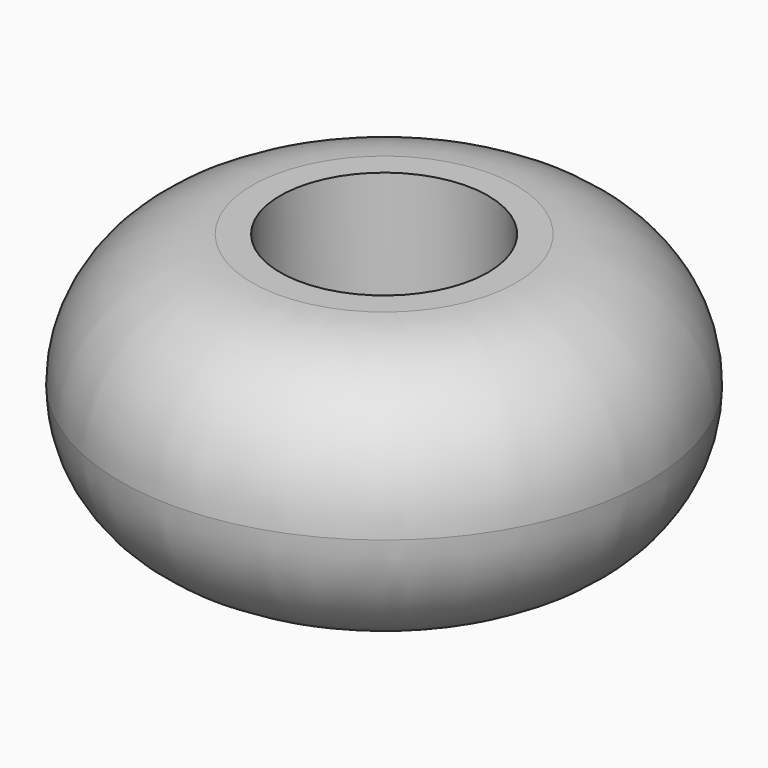
from build123d import *

# Parameters (mm, degrees)
F0_W     = 25.4
F0_H     = 25.4
F2_R     = 12.69999
F3_R     = 10
F4_DEPTH = 20.32
F5_R     = 10


# Not quite as in the source:
# - a fillet or chamfer is up to 0.001 mm smaller than in the source, because OpenCascade refuses the exact size


with BuildPart() as f1:
    # F0 (on Front) → F1 (revolve)
    with BuildSketch(Plane.XZ):
        with Locations((12.7, 12.7)):
            Rectangle(F0_W, F0_H)
    revolve(axis=Axis((0, 0, 17.3243917525), (0, 0, 1)))

    # F2 (radius 12.7 in the source; OpenCascade refuses exactly that, so slightly less here)
    f2_edges = [f1.edges().sort_by_distance(p)[0] for p in [
        (-25.4, 0, 0),
        (-25.4, 0, 25.4),
        (25.4, 0, 12.7),
    ]]
    fillet(f2_edges, radius=F2_R)

    # F3 (on face) → F4 (cut)
    with BuildSketch(Plane.XY.offset(25.4)):
        Circle(F3_R)
    extrude(amount=-F4_DEPTH, mode=Mode.SUBTRACT)

    # F5
    f5_edges = [f1.edges().sort_by_distance(p)[0] for p in [
        (-10, 0, 5.08),
    ]]
    fillet(f5_edges, radius=F5_R)


solid = f1.part
